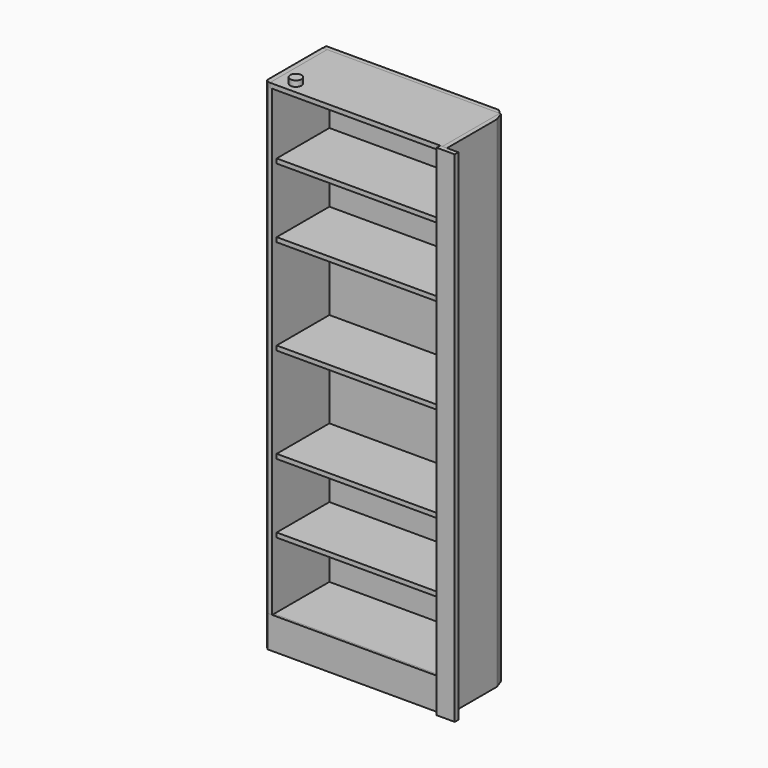
from build123d import *

# Parameters (mm, degrees)
F0_W           = 350
F0_H           = 2200
F1_DEPTH       = 15
F5_W           = 760
F5_H           = 350
F6_DEPTH       = 20
F7_W           = 760
F7_H           = 350
F8_DEPTH       = 20
F29_W          = 800
F29_H          = 10
F30_DEPTH      = 140
F34_W          = 80
F34_H          = 20
F35_DEPTH      = 1100
F35_DEPTH_BACK = 1100
F36_R          = 25
F37_DEPTH      = 25
F40_W          = 820.3160464764
F40_H          = 60
F41_DEPTH      = 1100
F41_DEPTH_BACK = 1100
F44_W          = 781.2406718731
F44_H          = 612.3302876949
F45_DEPTH      = 20
F44_W_2        = 782.2826504707
F44_H_2        = 1164.5840704441
F47_W          = 781.5454006195
F47_H          = 415.5381992459
F48_DEPTH      = 20
F50_SIZE2      = 19.99999
F50_SIZE       = 19.99999
F50_2_SIZE2    = 19.99999
F50_2_SIZE     = 19.99999
F50_3_SIZE2    = 19.99999
F50_3_SIZE     = 19.99999
F52_SIZE2      = 14.5588093706
F52_SIZE       = 40
F53_SIZE2      = 9.99999
F53_SIZE       = 9.99999
F53_2_SIZE2    = 9.99999
F53_2_SIZE     = 9.99999


# Not quite as in the source:
# - a fillet or chamfer is up to 0.001 mm smaller than in the source, because OpenCascade refuses the exact size


with BuildPart() as f1:
    # F0 (on Right) → F1 (new body, symmetric)
    with BuildSketch(Plane.YZ):
        Rectangle(F0_W, F0_H)
    extrude(amount=F1_DEPTH, both=True)


with BuildPart() as f2_1:
    # F2: copy of F1
    add(f1.part.moved(Location((-740, 0, 0))))


with BuildPart() as f2_1_1:
    # F3: moved
    add(f2_1.part.moved(Location((-30, 0, 0))))


with BuildPart() as f1_1:
    # F4: moved
    add(f1.part.moved(Location((385, 0, 0))))


with BuildPart() as f2_1_2:
    # F4: moved
    add(f2_1_1.part.moved(Location((385, 0, 0))))


with BuildPart() as f6:
    # F5 (on Top) → F6 (new body)
    with BuildSketch(Plane.XY):
        Rectangle(F5_W, F5_H)
    extrude(amount=F6_DEPTH)


with BuildPart() as f8:
    # F7 (on Top) → F8 (new body)
    with BuildSketch(Plane.XY):
        Rectangle(F7_W, F7_H)
    extrude(amount=F8_DEPTH)


with BuildPart() as f8_1:
    # F9: moved
    add(f8.part.moved(Location((0, 0, -980))))


with BuildPart() as f8_2:
    # F10: moved
    add(f8_1.part.moved(Location((0, 0, 300))))


with BuildPart() as f8_3:
    # F11: moved
    add(f8_2.part.moved(Location((0, 0, 400))))


with BuildPart() as f8_4:
    # F12: moved
    add(f8_3.part.moved(Location((0, 0, 300))))


with BuildPart() as f8_5:
    # F13: moved
    add(f8_4.part.moved(Location((0, 0, 300))))


with BuildPart() as f8_6:
    # F14: moved
    add(f8_5.part.moved(Location((0, 0, 400))))


with BuildPart() as f8_7:
    # F15: moved
    add(f8_6.part.moved(Location((0, 0, 360))))


with BuildPart() as f16_1:
    # F16: copy of F8
    add(f8_7.part.moved(Location((0, 0, -2060))))


with BuildPart() as f6_1:
    # F17: moved
    add(f6.part.moved(Location((0, 25, 779.46))))


with BuildPart() as f1_2:
    add(f1_1.part)

    # F18: cut F8
    add(f8_7.part, mode=Mode.SUBTRACT)

    # F19: cut F16_1
    add(f16_1.part, mode=Mode.SUBTRACT)

    # F20: cut F6
    add(f6_1.part, mode=Mode.SUBTRACT)


with BuildPart() as f2_1_3:
    add(f2_1_2.part)

    # F18: cut F8
    add(f8_7.part, mode=Mode.SUBTRACT)

    # F19: cut F16_1
    add(f16_1.part, mode=Mode.SUBTRACT)

    # F20: cut F6
    add(f6_1.part, mode=Mode.SUBTRACT)


with BuildPart() as f21_1:
    # F21: copy of F6
    add(f6_1.part.moved(Location((0, 0, -305))))


with BuildPart() as f2_1_4:
    add(f2_1_3.part)

    # F22: cut F21_1
    add(f21_1.part, mode=Mode.SUBTRACT)


with BuildPart() as f1_3:
    add(f1_2.part)

    # F22: cut F21_1
    add(f21_1.part, mode=Mode.SUBTRACT)


with BuildPart() as f23_1:
    # F23: copy of F21_1
    add(f21_1.part.moved(Location((0, 0, -420))))


with BuildPart() as f2_1_5:
    add(f2_1_4.part)

    # F24: cut F23_1
    add(f23_1.part, mode=Mode.SUBTRACT)


with BuildPart() as f1_4:
    add(f1_3.part)

    # F24: cut F23_1
    add(f23_1.part, mode=Mode.SUBTRACT)


with BuildPart() as f25_1:
    # F25: copy of F23_1
    add(f23_1.part.moved(Location((0, 0, -420))))


with BuildPart() as f1_5:
    add(f1_4.part)

    # F26: cut F25_1
    add(f25_1.part, mode=Mode.SUBTRACT)


with BuildPart() as f2_1_6:
    add(f2_1_5.part)

    # F26: cut F25_1
    add(f25_1.part, mode=Mode.SUBTRACT)


with BuildPart() as f27_1:
    # F27: copy of F25_1
    add(f25_1.part.moved(Location((0, 0, -305))))


with BuildPart() as f1_6:
    add(f1_5.part)

    # F28: cut F27_1
    add(f27_1.part, mode=Mode.SUBTRACT)


with BuildPart() as f2_1_7:
    add(f2_1_6.part)

    # F28: cut F27_1
    add(f27_1.part, mode=Mode.SUBTRACT)


with BuildPart() as f30:
    # F29 (on Top) → F30 (new body)
    with BuildSketch(Plane.XY):
        with Locations((-0.3543496132, -205.0241075132)):
            Rectangle(F29_W, F29_H)
    extrude(amount=F30_DEPTH)


with BuildPart() as f30_1:
    # F31: moved
    add(f30.part.moved(Location((0, 15.02, -1100))))


with BuildPart() as f30_2:
    # F32: moved
    add(f30_1.part.moved(Location((0, 20, 0))))


with BuildPart() as f1_7:
    add(f1_6.part)

    # F33: cut F30
    add(f30_2.part, mode=Mode.SUBTRACT)


with BuildPart() as f2_1_8:
    add(f2_1_7.part)

    # F33: cut F30
    add(f30_2.part, mode=Mode.SUBTRACT)


with BuildPart() as f16_1_1:
    add(f16_1.part)

    # F33: cut F30
    add(f30_2.part, mode=Mode.SUBTRACT)


with BuildPart() as f35:
    # F34 (on Top) → F35 (new body, two sides)
    with BuildSketch(Plane.XY) as f35_sk:
        with Locations((370.0484473851, -209.9858894944)):
            Rectangle(F34_W, F34_H)
    extrude(amount=F35_DEPTH)
    extrude(f35_sk.sketch, amount=-F35_DEPTH_BACK)


with BuildPart() as f37:
    # F36 (on Top) → F37 (new body)
    with BuildSketch(Plane.XY):
        with Locations((-335.9403908253, -154.3275415897)):
            Circle(F36_R)
    extrude(amount=F37_DEPTH)


with BuildPart() as f37_1:
    # F38: moved
    add(f37.part.moved(Location((30, 30, 1100))))


with BuildPart() as f35_1:
    # F39: moved
    add(f35.part.moved(Location((40, 25, 0))))


with BuildPart() as f41:
    # F40 (on Top) → F41 (new body, two sides)
    with BuildSketch(Plane.XY) as f41_sk:
        with Locations((7.9502910376, 92.0613843203)):
            Rectangle(F40_W, F40_H)
    extrude(amount=F41_DEPTH)
    extrude(f41_sk.sketch, amount=-F41_DEPTH_BACK)


with BuildPart() as f41_1:
    # F42: moved
    add(f41.part.moved(Location((-8, 78, 0))))


with BuildPart() as f1_8:
    add(f1_7.part)

    # F43: cut F41
    add(f41_1.part, mode=Mode.SUBTRACT)

    # F51: cut F30
    add(f30_2.part, mode=Mode.SUBTRACT)

    # F52
    f52_edges = [f1_8.edges().sort_by_distance(p)[0] for p in [
        (400, 140.061384, 0),
    ]]
    f52_side = f1_8.faces().sort_by_distance((400, -17.469308, 0))[0]
    chamfer(f52_edges, length=F52_SIZE, length2=F52_SIZE2, reference=f52_side)


with BuildPart() as f2_1_9:
    add(f2_1_8.part)

    # F43: cut F41
    add(f41_1.part, mode=Mode.SUBTRACT)

    # F51: cut F30
    add(f30_2.part, mode=Mode.SUBTRACT)

    # F53 (size 10 and 10 in the source; OpenCascade refuses exactly that, so slightly less here)
    f53_edges = [f2_1_9.edges().sort_by_distance(p)[0] for p in [
        (-400, -175, 70),
    ]]
    chamfer(f53_edges, length=F53_SIZE, length2=F53_SIZE2)


with BuildPart() as f6_2:
    add(f6_1.part)

    # F43: cut F41
    add(f41_1.part, mode=Mode.SUBTRACT)


with BuildPart() as f8_8:
    add(f8_7.part)

    # F43: cut F41
    add(f41_1.part, mode=Mode.SUBTRACT)


with BuildPart() as f16_1_2:
    add(f16_1_1.part)

    # F43: cut F41
    add(f41_1.part, mode=Mode.SUBTRACT)

    # F51: cut F30
    add(f30_2.part, mode=Mode.SUBTRACT)


with BuildPart() as f21_1_1:
    add(f21_1.part)

    # F43: cut F41
    add(f41_1.part, mode=Mode.SUBTRACT)


with BuildPart() as f23_1_1:
    add(f23_1.part)

    # F43: cut F41
    add(f41_1.part, mode=Mode.SUBTRACT)


with BuildPart() as f25_1_1:
    add(f25_1.part)

    # F43: cut F41
    add(f41_1.part, mode=Mode.SUBTRACT)


with BuildPart() as f27_1_1:
    add(f27_1.part)

    # F43: cut F41
    add(f41_1.part, mode=Mode.SUBTRACT)


with BuildPart() as f45:
    # F44 (on Front) → F45 (new body)
    with BuildSketch(Plane.XZ):
        with Locations((-9.511962533, 792.8916960955)):
            Rectangle(F44_W, F44_H)
    extrude(amount=F45_DEPTH)


with BuildPart() as f45b:
    # F44 (on Front) → F45, piece 2 (new body)
    with BuildSketch(Plane.XZ):
        with Locations((-9.7425580025, -517.82540977)):
            Rectangle(F44_W_2, F44_H_2)
    extrude(amount=F45_DEPTH)


with BuildPart() as f45_1:
    # F46: moved
    add(f45.part.moved(Location((0, 160, 0))))

    # F50 (size 20 and 20 in the source; OpenCascade refuses exactly that, so slightly less here)
    f50_edges = [f45_1.edges().sort_by_distance(p)[0] for p in [
        (381.108373, 160, 792.891696),
    ]]
    chamfer(f50_edges, length=F50_SIZE, length2=F50_SIZE2)


with BuildPart() as f45b_1:
    # F46: moved
    add(f45b.part.moved(Location((0, 160, 0))))

    # F50#3 (size 20 and 20 in the source; OpenCascade refuses exactly that, so slightly less here)
    f50_3_edges = [f45b_1.edges().sort_by_distance(p)[0] for p in [
        (381.398767, 160, -517.82541),
    ]]
    chamfer(f50_3_edges, length=F50_3_SIZE, length2=F50_3_SIZE2)


with BuildPart() as f48:
    # F47 (on Front) → F48 (new body)
    with BuildSketch(Plane.XZ):
        with Locations((-9.801954031, 274.3636928499)):
            Rectangle(F47_W, F47_H)
    extrude(amount=F48_DEPTH)


with BuildPart() as f48_1:
    # F49: moved
    add(f48.part.moved(Location((0, 160, 0))))

    # F50#2 (size 20 and 20 in the source; OpenCascade refuses exactly that, so slightly less here)
    f50_2_edges = [f48_1.edges().sort_by_distance(p)[0] for p in [
        (380.970746, 160, 274.363693),
    ]]
    chamfer(f50_2_edges, length=F50_2_SIZE, length2=F50_2_SIZE2)


with BuildPart() as f30_3:
    add(f30_2.part)

    # F53#2 (size 10 and 10 in the source; OpenCascade refuses exactly that, so slightly less here)
    f53_2_edges = [f30_3.edges().sort_by_distance(p)[0] for p in [
        (-400.35435, -175.004108, -1030),
    ]]
    chamfer(f53_2_edges, length=F53_2_SIZE, length2=F53_2_SIZE2)


with BuildPart() as f54_1:
    # F54: copy of F16_1
    add(f16_1_2.part.moved(Location((0, 0, -20))))


with BuildPart() as f2_1_10:
    add(f2_1_9.part)

    # F55: cut F54_1
    add(f54_1.part, mode=Mode.SUBTRACT)


with BuildPart() as f1_9:
    add(f1_8.part)

    # F55: cut F54_1
    add(f54_1.part, mode=Mode.SUBTRACT)


solid = Compound([f37_1.part, f35_1.part, f6_2.part, f8_8.part, f16_1_2.part, f21_1_1.part, f23_1_1.part, f25_1_1.part, f27_1_1.part, f45_1.part, f45b_1.part, f48_1.part, f30_3.part, f54_1.part, f2_1_10.part, f1_9.part])
